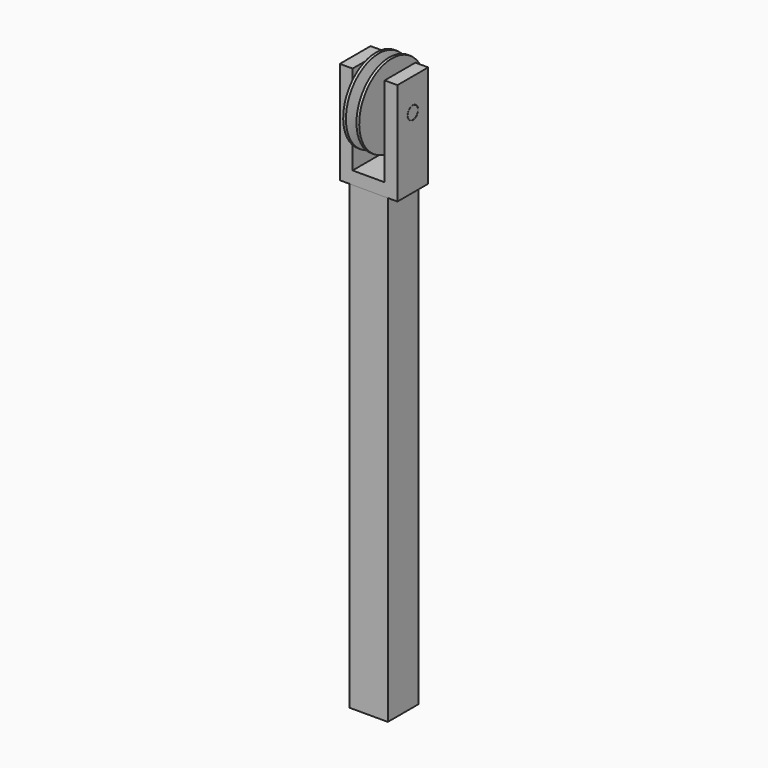
from build123d import *

# Parameters (mm, degrees)
F3_DEPTH      = 19.05
F4_R          = 6.50875
F5_DEPTH      = 28.576
F5_DEPTH_BACK = 28.576
F6_W          = 38.1
F6_H          = 38.1
F7_DEPTH      = 457.2
F8_R          = 6.35
F9_DEPTH      = 57.15


with BuildPart() as f1:
    # F0 (on Front) → F1 (revolve)
    with BuildSketch(Plane.XZ):
        Polygon((0, 6.35), (0, 22.225), (-1.984375, 22.225), (-5.2314363497, 40.64), (-7.9375, 40.64), (-7.9375, 6.35), align=None)
        Polygon((1.984375, 22.225), (0, 22.225), (0, 6.35), (7.9375, 6.35), (7.9375, 40.64), (5.2314363497, 40.64), align=None)
    revolve(axis=Axis((0, 0, 0), (1, 0, 0)))

    # F8 (on face) → F9 (join)
    with BuildSketch(Plane.YZ.offset(28.575)):
        Circle(F8_R)
    extrude(amount=-F9_DEPTH)


with BuildPart() as f3:
    # F2 (on Front) → F3 (new body, symmetric)
    with BuildSketch(Plane.XZ):
        Polygon((28.575, -69.85), (28.575, 31.75), (15.875, 31.75), (15.875, -57.15), (-15.875, -57.15), (-15.875, 31.75), (-28.575, 31.75), (-28.575, -69.85), align=None)
    extrude(amount=F3_DEPTH, both=True)

    # F4 (on Right) → F5 (cut, two sides)
    with BuildSketch(Plane.YZ) as f5_sk:
        Circle(F4_R)
    extrude(amount=-F5_DEPTH, mode=Mode.SUBTRACT)
    extrude(f5_sk.sketch, amount=F5_DEPTH_BACK, mode=Mode.SUBTRACT)


with BuildPart() as f7:
    # F6 (on face) → F7 (new body)
    with BuildSketch(Plane(origin=(0, 0, -69.85), x_dir=(1, 0, 0), z_dir=(0, 0, -1))):
        Rectangle(F6_W, F6_H)
    extrude(amount=F7_DEPTH)


solid = Compound([f1.part, f3.part, f7.part])
